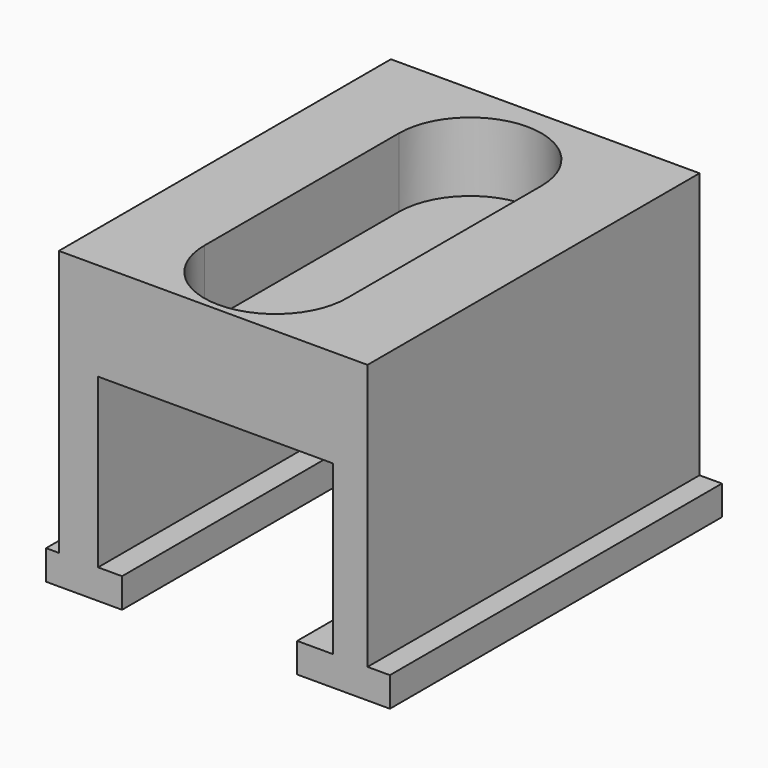
from build123d import *

# Parameters (mm, degrees)
F1_DEPTH = 152.4
F2_W     = 113.335262984
F2_H     = 152.4
F3_DEPTH = 25.4


# Not quite as in the source:
# - a feature names something its author has since deleted; it is built from what else it names


with BuildPart() as f1:
    # F0 (on Front) → F1 (new body)
    with BuildSketch(Plane.XZ):
        Polygon((-61.8058890104, -21.7274855822), (-66.5037259459, -21.7274855822), (-66.5037259459, -32.5912311673), (-38.6103317142, -32.5912311673), (-38.6103317142, -21.7274855822), (-47.4187731743, -21.7274855822), (-47.4187731743, 39.9315953255), (38.9039441943, 39.9315953255), (38.9039441943, -21.7274855822), (25.6912820041, -21.7274855822), (25.6912820041, -32.5912311673), (59.7505830228, -32.5912311673), (59.7505830228, -21.7274855822), (51.5293739736, -21.7274855822), (51.5293739736, 50.5017265677), (-61.8058890104, 50.5017265677), align=None)
    extrude(amount=F1_DEPTH)

    # F2 (on face) → F3 (join)
    with BuildSketch(Plane.XY.offset(50.5017265677)):
        with Locations((-5.1382575184, -76.2)):
            Rectangle(F2_W, F2_H)
        with BuildLine():
            Line((-31.2988758087, -123.7941682339), (-31.2988758087, -34.4304777682))
            ThreePointArc((-31.2988758087, -34.4304777682), (-5.1382575184, -8.2698594779), (21.0223607719, -34.4304777682))
            Line((21.0223607719, -34.4304777682), (21.0223607719, -123.7941682339))
            ThreePointArc((21.0223607719, -123.7941682339), (-5.1382575184, -149.9547865242), (-31.2988758087, -123.7941682339))
        make_face(mode=Mode.SUBTRACT)
    extrude(amount=F3_DEPTH)


solid = f1.part
